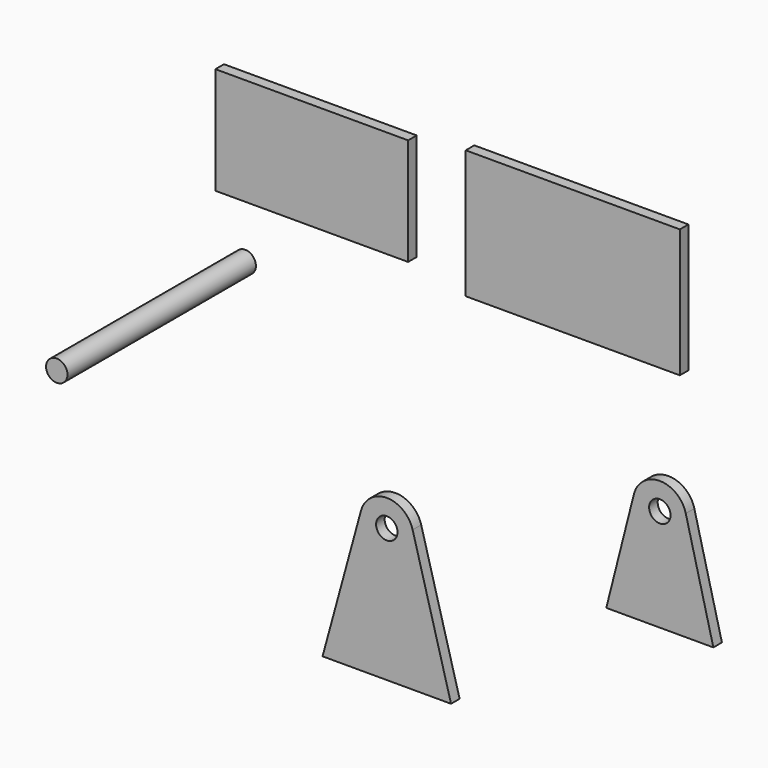
from build123d import *

# Parameters (mm, degrees)
F0_W     = 40
F0_H     = 24
F1_DEPTH = 2
F2_R     = 2
F3_DEPTH = 2
F4_R     = 2
F5_DEPTH = 44
F6_W     = 36
F6_H     = 20
F7_DEPTH = 2
F8_R     = 2
F9_DEPTH = 2


# Not quite as in the source:
# - a feature of the source that left no trace in its solid (it failed there, or was rolled back) is left out


with BuildPart() as f1:
    # F0 (on Front) → F1 (new body)
    with BuildSketch(Plane.XZ):
        with Locations((-2.604843583, -6.1964805115)):
            Rectangle(F0_W, F0_H)
    extrude(amount=F1_DEPTH)


with BuildPart() as f3:
    # F2 (on Front) → F3 (new body)
    with BuildSketch(Plane.XZ):
        with BuildLine():
            Line((-42.1746947658, -59.8358749318), (-49.3476256423, -86.1108493255))
            Line((-49.3476256423, -86.1108493255), (-25.3476256423, -86.1108493255))
            Line((-25.3476256423, -86.1108493255), (-32.5205565188, -59.8358749318))
            ThreePointArc((-32.5205565188, -59.8358749318), (-32.3882734917, -60.4888642222), (-32.3439170108, -61.1536396093))
            ThreePointArc((-32.3439170108, -61.1536396093), (-38.0124010294, -66.1129917599), (-42.1746947658, -59.8358749318))
        make_face()
        with BuildLine():
            ThreePointArc((-32.5205565188, -59.8358749318), (-37.3476256423, -56.1499309779), (-42.1746947658, -59.8358749318))
            ThreePointArc((-42.1746947658, -59.8358749318), (-38.0124010294, -66.1129917599), (-32.3439170108, -61.1536396093))
            ThreePointArc((-32.3439170108, -61.1536396093), (-32.3882734917, -60.4888642222), (-32.5205565188, -59.8358749318))
        make_face()
        with Locations((-37.3476256423, -61.1536396093)):
            Circle(F2_R, mode=Mode.SUBTRACT)
    extrude(amount=F3_DEPTH)


with BuildPart() as f5:
    # F4 (on Front) → F5 (new body)
    with BuildSketch(Plane.XZ):
        with Locations((-65.3979107738, -27.2803399712)):
            Circle(F4_R)
    extrude(amount=F5_DEPTH)


with BuildPart() as f7:
    # F6 (on Front) → F7 (new body)
    with BuildSketch(Plane.XZ):
        with Locations((-51.3647299066, -6.0609190166)):
            Rectangle(F6_W, F6_H)
    extrude(amount=F7_DEPTH)


with BuildPart() as f9:
    # F8 (on Front) → F9 (new body)
    with BuildSketch(Plane.XZ):
        with BuildLine():
            Line((8.8063688133, -40.5499661908), (3.6535110436, -60.907963558))
            Line((3.6535110436, -60.907963558), (23.6535110436, -60.907963558))
            Line((23.6535110436, -60.907963558), (18.5006532739, -40.5499661908))
            ThreePointArc((18.5006532739, -40.5499661908), (18.6151494399, -41.1586587773), (18.6535110436, -41.7768370883))
            ThreePointArc((18.6535110436, -41.7768370883), (13.0353327326, -46.7384754847), (8.8063688133, -40.5499661908))
        make_face()
        with BuildLine():
            ThreePointArc((18.5006532739, -40.5499661908), (13.6535110436, -36.7768370883), (8.8063688133, -40.5499661908))
            ThreePointArc((8.8063688133, -40.5499661908), (13.0353327326, -46.7384754847), (18.6535110436, -41.7768370883))
            ThreePointArc((18.6535110436, -41.7768370883), (18.6151494399, -41.1586587773), (18.5006532739, -40.5499661908))
        make_face()
        with Locations((13.6535110436, -41.7768370883)):
            Circle(F8_R, mode=Mode.SUBTRACT)
    extrude(amount=F9_DEPTH)


solid = Compound([f1.part, f3.part, f5.part, f7.part, f9.part])
